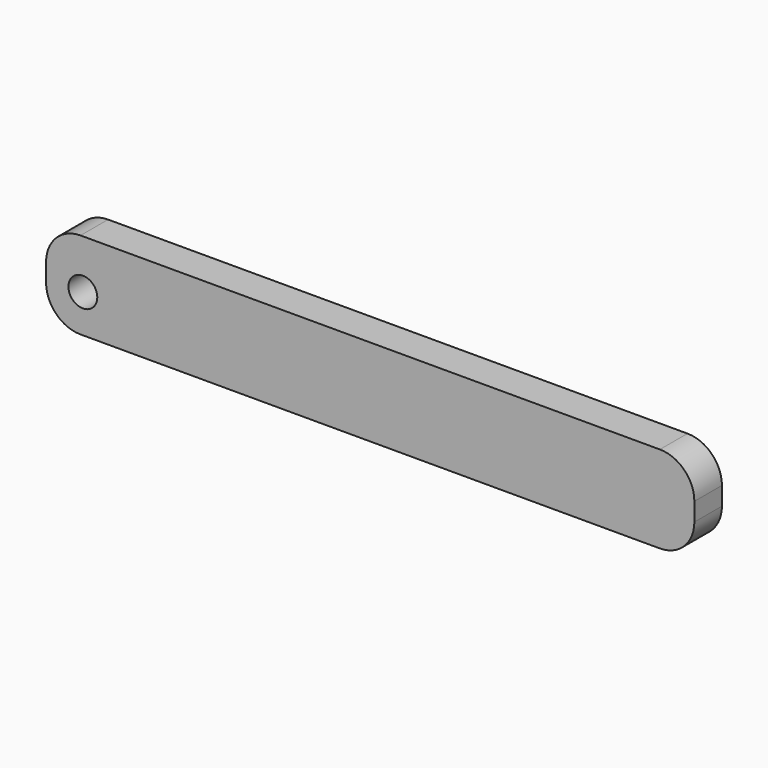
from build123d import *

# Parameters (mm, degrees)
F0_W     = 94.0563417971
F0_H     = 12.6443672925
F0_R     = 2.0927521529
F1_DEPTH = 5
F2_R     = 5


# Not quite as in the source:
# - the program builds the solid bodies; features that only make, move or delete a surface that nothing else refers to are left out


with BuildPart() as f1:
    # F0 (on Front) → F1 (new body)
    with BuildSketch(Plane.XZ):
        with Locations((-9.9823940545, 22.7376772091)):
            Rectangle(F0_W, F0_H)
        with Locations((-51.6735911369, 21.9417177141)):
            Circle(F0_R, mode=Mode.SUBTRACT)
    extrude(amount=F1_DEPTH)

    # F2
    f2_edges = [f1.edges().sort_by_distance(p)[0] for p in [
        (37.045777, -2.5, 29.059861),
        (37.045777, -2.5, 16.415494),
        (-57.010565, -2.5, 16.415494),
        (-57.010565, -2.5, 29.059861),
    ]]
    fillet(f2_edges, radius=F2_R)


solid = f1.part
